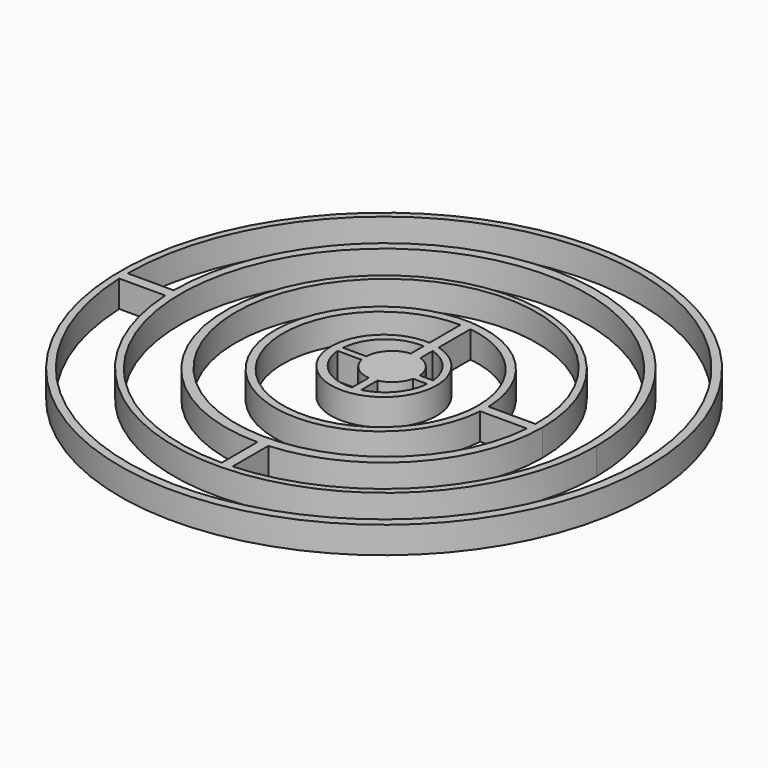
from build123d import *

# Parameters (mm, degrees)
F0_R      = 250
F0_R_2    = 242.5
F6_DEPTH  = 25.4
F1_R      = 200
F1_R_2    = 192.5
F7_DEPTH  = 25.4
F2_R      = 150
F2_R_2    = 142.5
F8_DEPTH  = 25.4
F3_R      = 100
F3_R_2    = 92.5
F9_DEPTH  = 25.4
F4_R      = 50
F4_R_2    = 42.5
F10_DEPTH = 25.4
F5_R      = 25
F11_DEPTH = 25.4
F12_W     = 53.4157007933
F12_H     = 10.408022441
F12_W_2   = 10.0719733164
F12_H_2   = 50.3633767366
F12_W_3   = 52.6525899768
F12_H_3   = 9.6449414268
F12_H_4   = 41.9694781303
F12_H_5   = 22.8924434632
F12_W_4   = 30.523262918
F12_H_6   = 6.3797682524
F12_W_5   = 17.5508763641
F12_H_7   = 7.1428497322
F12_W_6   = 7.7827312052
F12_H_8   = 28.9970943704
F13_DEPTH = 25.4


with BuildPart() as f6:
    # F0 (on Top) → F6 (new body)
    with BuildSketch(Plane.XY):
        with Locations((-0.2296342573, -0.8695026627)):
            Circle(F0_R)
        with Locations((-1.2017333358, -0.1394655317)):
            Circle(F0_R_2, mode=Mode.SUBTRACT)
    extrude(amount=F6_DEPTH)



with BuildPart() as f7:
    # F1 (on Top) → F7 (new body)
    with BuildSketch(Plane.XY):
        with Locations((-0.229648911, 0.6240262301)):
            Circle(F1_R)
        with Locations((-0.229648911, -0.9403247815)):
            Circle(F1_R_2, mode=Mode.SUBTRACT)
    extrude(amount=F7_DEPTH)


with BuildPart() as f8:
    # F2 (on Top) → F8 (new body)
    with BuildSketch(Plane.XY):
        with Locations((-0.0088901297, -1.2084672926)):
            Circle(F2_R)
        with Locations((-0.0048156621, 1.2250516324)):
            Circle(F2_R_2, mode=Mode.SUBTRACT)
    extrude(amount=F8_DEPTH)


with BuildPart() as f9:
    # F3 (on Top) → F9 (new body)
    with BuildSketch(Plane.XY):
        with Locations((-1.9242773997, -2.7173017152)):
            Circle(F3_R)
        with Locations((-1.5612963189, -3.2658300582)):
            Circle(F3_R_2, mode=Mode.SUBTRACT)
    extrude(amount=F9_DEPTH)


with BuildPart() as f10:
    # F4 (on Top) → F10 (new body)
    with BuildSketch(Plane.XY):
        with Locations((-3.2166936435, 2.6153912768)):
            Circle(F4_R)
        with Locations((-2.5570748915, 3.2750012369)):
            Circle(F4_R_2, mode=Mode.SUBTRACT)
    extrude(amount=F10_DEPTH)


with BuildPart() as f11:
    # F5 (on Top) → F11 (new body)
    with BuildSketch(Plane.XY):
        with Locations((2.1465087775, 5.5706012063)):
            Circle(F5_R)
    extrude(amount=F11_DEPTH)


with BuildPart() as f6_1:
    add(f6.part)

    add(f7.part)  # F13 merges F7

    add(f8.part)  # F13 merges F8

    add(f9.part)  # F13 merges F9

    add(f10.part)  # F13 merges F10

    add(f11.part)  # F13 merges F11
    # F12 (on face) → F13 (join)
    with BuildSketch(Plane.XY):
        with Locations((-222.6678654552, -5.2040112205)):
            Rectangle(F12_W, F12_H)
        with Locations((5.0359866582, -172.9443594813)):
            Rectangle(F12_W_2, F12_H_2)
        with Locations((121.1003102362, -4.8224707134)):
            Rectangle(F12_W_3, F12_H_3)
        with Locations((5.0359866582, 70.097066462)):
            Rectangle(F12_W_2, F12_H_4)
        with Locations((5.0359866582, 37.6661056653)):
            Rectangle(F12_W_2, F12_H_5)
        with Locations((-31.8975038826, 3.1898841262)):
            Rectangle(F12_W_4, F12_H_6)
        with Locations((34.8721230403, 3.5714248661)):
            Rectangle(F12_W_5, F12_H_7)
        with Locations((3.8913656026, -27.9588955455)):
            Rectangle(F12_W_6, F12_H_8)
    extrude(amount=F13_DEPTH)


solid = f6_1.part
